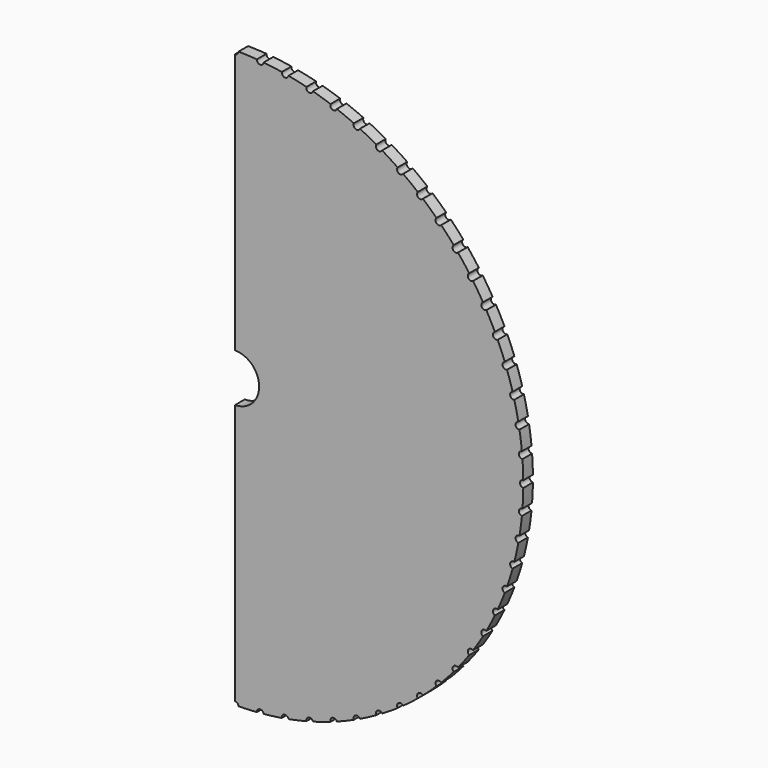
from build123d import *

# Parameters (mm, degrees)
F2_DEPTH = 3.175
F3_D     = 12.7


with BuildPart() as f2:
    # F0 (on Front) → F2 (new body)
    with BuildSketch(Plane.XZ):
        with BuildLine():
            ThreePointArc((5.7552136035, 75.9823500319), (3.3237973172, 76.1274744845), (0.8889848745, 76.1948141667))
            ThreePointArc((0.8889848745, 76.1948141667), (0.6267817779, 75.5695512686), (0, 75.311))
            Line((0, 75.311), (0, -75.311))
            ThreePointArc((0, -75.311), (0.6267817779, -75.5695512686), (0.8889848745, -76.1948141667))
            ThreePointArc((0.8889848745, -76.1948141667), (3.3237973172, -76.1274744845), (5.7552136035, -75.9823500319))
            ThreePointArc((5.7552136035, -75.9823500319), (6.5637861421, -75.024418908), (7.5264176409, -75.8273897579))
            ThreePointArc((7.5264176409, -75.8273897579), (9.9460958472, -75.5480984367), (12.355611431, -75.1916143341))
            ThreePointArc((12.355611431, -75.1916143341), (13.0776179083, -74.1668566871), (14.1065698245, -74.8828731272))
            ThreePointArc((14.1065698245, -74.8828731272), (16.4926985821, -74.3937557425), (18.8619755949, -73.8286250492))
            ThreePointArc((18.8619755949, -73.8286250492), (19.4919211057, -72.7448399037), (20.5793624939, -73.3684526165))
            ThreePointArc((20.5793624939, -73.3684526165), (22.9137819222, -72.673231647), (25.2247887354, -71.9037553488))
            ThreePointArc((25.2247887354, -71.9037553488), (25.757879014, -70.769190964), (26.8955337885, -71.2956538804))
            ThreePointArc((26.8955337885, -71.2956538804), (29.1604775462, -70.3996203774), (31.3956260024, -69.4316546534))
            ThreePointArc((31.3956260024, -69.4316546534), (31.82780391, -68.2549457495), (33.0070138311, -68.6802521687))
            ThreePointArc((33.0070138311, -68.6802521687), (35.1852443285, -67.5902254882), (37.3275235984, -66.4311371422))
            ThreePointArc((37.3275235984, -66.4311371422), (37.6555, -65.2212391844), (38.8672905683, -65.5421522677))
            ThreePointArc((38.8672905683, -65.5421522677), (40.942230156, -64.2664281709), (42.9753362008, -62.9250385651))
            ThreePointArc((42.9753362008, -62.9250385651), (43.196614998, -61.6911596074), (44.4317637555, -61.9052370125))
            ThreePointArc((44.4317637555, -61.9052370125), (46.3876208905, -60.4535245302), (48.2960805456, -58.9400424494))
            ThreePointArc((48.2960805456, -58.9400424494), (48.4089776731, -57.6915730557), (49.6580843918, -57.7971855243))
            ThreePointArc((49.6580843918, -57.7971855243), (51.4799738203, -56.1805330649), (53.2492625554, -54.5064770216))
            ThreePointArc((53.2492625554, -54.5064770216), (53.2529187979, -53.2529187979), (54.5064770216, -53.2492625554))
            ThreePointArc((54.5064770216, -53.2492625554), (56.1805330649, -51.4799738203), (57.7971855243, -49.6580843918))
            ThreePointArc((57.7971855243, -49.6580843918), (57.6915730557, -48.4089776731), (58.9400424494, -48.2960805456))
            ThreePointArc((58.9400424494, -48.2960805456), (60.4535245302, -46.3876208905), (61.9052370125, -44.4317637555))
            ThreePointArc((61.9052370125, -44.4317637555), (61.6911596074, -43.196614998), (62.9250385651, -42.9753362008))
            ThreePointArc((62.9250385651, -42.9753362008), (64.2664281709, -40.942230156), (65.5421522677, -38.8672905683))
            ThreePointArc((65.5421522677, -38.8672905683), (65.2212391844, -37.6555), (66.4311371422, -37.3275235984))
            ThreePointArc((66.4311371422, -37.3275235984), (67.5902254882, -35.1852443285), (68.6802521687, -33.0070138311))
            ThreePointArc((68.6802521687, -33.0070138311), (68.2549457495, -31.82780391), (69.4316546534, -31.3956260024))
            ThreePointArc((69.4316546534, -31.3956260024), (70.3996203774, -29.1604775462), (71.2956538804, -26.8955337885))
            ThreePointArc((71.2956538804, -26.8955337885), (70.769190964, -25.757879014), (71.9037553488, -25.2247887354))
            ThreePointArc((71.9037553488, -25.2247887354), (72.673231647, -22.9137819222), (73.3684526165, -20.5793624939))
            ThreePointArc((73.3684526165, -20.5793624939), (72.7448399037, -19.4919211057), (73.8286250492, -18.8619755949))
            ThreePointArc((73.8286250492, -18.8619755949), (74.3937557425, -16.4926985821), (74.8828731272, -14.1065698245))
            ThreePointArc((74.8828731272, -14.1065698245), (74.1668566871, -13.0776179083), (75.1916143341, -12.355611431))
            ThreePointArc((75.1916143341, -12.355611431), (75.5480984367, -9.9460958472), (75.8273897579, -7.5264176409))
            ThreePointArc((75.8273897579, -7.5264176409), (75.024418908, -6.5637861421), (75.9823500319, -5.7552136035))
            ThreePointArc((75.9823500319, -5.7552136035), (76.1274744845, -3.3237973172), (76.1948141667, -0.8889848745))
            ThreePointArc((76.1948141667, -0.8889848745), (75.311, 0), (76.1948141667, 0.8889848745))
            ThreePointArc((76.1948141667, 0.8889848745), (76.1274744845, 3.3237973172), (75.9823500319, 5.7552136035))
            ThreePointArc((75.9823500319, 5.7552136035), (75.024418908, 6.5637861421), (75.8273897579, 7.5264176409))
            ThreePointArc((75.8273897579, 7.5264176409), (75.5480984367, 9.9460958472), (75.1916143341, 12.355611431))
            ThreePointArc((75.1916143341, 12.355611431), (74.1668566871, 13.0776179083), (74.8828731272, 14.1065698245))
            ThreePointArc((74.8828731272, 14.1065698245), (74.3937557425, 16.4926985821), (73.8286250492, 18.8619755949))
            ThreePointArc((73.8286250492, 18.8619755949), (72.7448399037, 19.4919211057), (73.3684526165, 20.5793624939))
            ThreePointArc((73.3684526165, 20.5793624939), (72.673231647, 22.9137819222), (71.9037553488, 25.2247887354))
            ThreePointArc((71.9037553488, 25.2247887354), (70.769190964, 25.757879014), (71.2956538804, 26.8955337885))
            ThreePointArc((71.2956538804, 26.8955337885), (70.3996203774, 29.1604775462), (69.4316546534, 31.3956260024))
            ThreePointArc((69.4316546534, 31.3956260024), (68.2549457495, 31.82780391), (68.6802521687, 33.0070138311))
            ThreePointArc((68.6802521687, 33.0070138311), (67.5902254882, 35.1852443285), (66.4311371422, 37.3275235984))
            ThreePointArc((66.4311371422, 37.3275235984), (65.2212391844, 37.6555), (65.5421522677, 38.8672905683))
            ThreePointArc((65.5421522677, 38.8672905683), (64.2664281709, 40.942230156), (62.9250385651, 42.9753362008))
            ThreePointArc((62.9250385651, 42.9753362008), (61.6911596074, 43.196614998), (61.9052370125, 44.4317637555))
            ThreePointArc((61.9052370125, 44.4317637555), (60.4535245302, 46.3876208905), (58.9400424494, 48.2960805456))
            ThreePointArc((58.9400424494, 48.2960805456), (57.6915730557, 48.4089776731), (57.7971855243, 49.6580843918))
            ThreePointArc((57.7971855243, 49.6580843918), (56.1805330649, 51.4799738203), (54.5064770216, 53.2492625554))
            ThreePointArc((54.5064770216, 53.2492625554), (53.2529187979, 53.2529187979), (53.2492625554, 54.5064770216))
            ThreePointArc((53.2492625554, 54.5064770216), (51.4799738203, 56.1805330649), (49.6580843918, 57.7971855243))
            ThreePointArc((49.6580843918, 57.7971855243), (48.4089776731, 57.6915730557), (48.2960805456, 58.9400424494))
            ThreePointArc((48.2960805456, 58.9400424494), (46.3876208905, 60.4535245302), (44.4317637555, 61.9052370125))
            ThreePointArc((44.4317637555, 61.9052370125), (43.196614998, 61.6911596074), (42.9753362008, 62.9250385651))
            ThreePointArc((42.9753362008, 62.9250385651), (40.942230156, 64.2664281709), (38.8672905683, 65.5421522677))
            ThreePointArc((38.8672905683, 65.5421522677), (37.6555, 65.2212391844), (37.3275235984, 66.4311371422))
            ThreePointArc((37.3275235984, 66.4311371422), (35.1852443285, 67.5902254882), (33.0070138311, 68.6802521687))
            ThreePointArc((33.0070138311, 68.6802521687), (31.82780391, 68.2549457495), (31.3956260024, 69.4316546534))
            ThreePointArc((31.3956260024, 69.4316546534), (29.1604775462, 70.3996203774), (26.8955337885, 71.2956538804))
            ThreePointArc((26.8955337885, 71.2956538804), (25.757879014, 70.769190964), (25.2247887354, 71.9037553488))
            ThreePointArc((25.2247887354, 71.9037553488), (22.9137819222, 72.673231647), (20.5793624939, 73.3684526165))
            ThreePointArc((20.5793624939, 73.3684526165), (19.4919211057, 72.7448399037), (18.8619755949, 73.8286250492))
            ThreePointArc((18.8619755949, 73.8286250492), (16.4926985821, 74.3937557425), (14.1065698245, 74.8828731272))
            ThreePointArc((14.1065698245, 74.8828731272), (13.0776179083, 74.1668566871), (12.355611431, 75.1916143341))
            ThreePointArc((12.355611431, 75.1916143341), (9.9460958472, 75.5480984367), (7.5264176409, 75.8273897579))
            ThreePointArc((7.5264176409, 75.8273897579), (6.5637861421, 75.024418908), (5.7552136035, 75.9823500319))
        make_face()
    extrude(amount=F2_DEPTH)

    # F3 (through all)
    with Locations(Plane(origin=(0, 0, 0), x_dir=(1, 0, 0), z_dir=(0, 1, 0))):
        with Locations((0, 0)):
            Hole(F3_D / 2)


solid = f2.part
